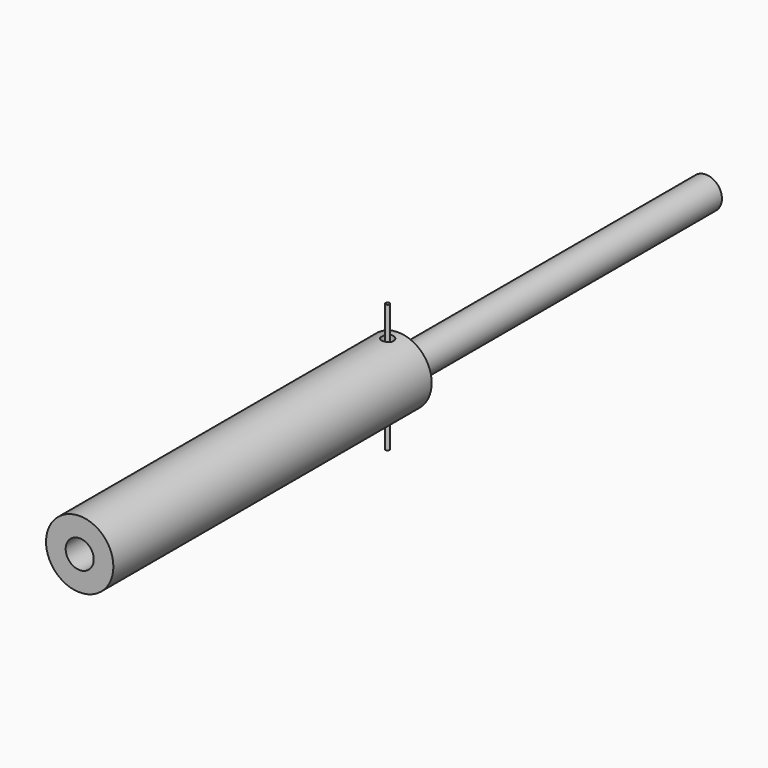
from build123d import *

# Parameters (mm, degrees)
F0_R      = 53.34
F0_R_2    = 22.225
F1_DEPTH  = 20.6375
F6_DEPTH  = 609.6
F5_R      = 9.525
F5_R_2    = 3.302
F7_DEPTH  = 19.05
F8_DEPTH  = 32.3616602869
F4_R      = 9.525
F4_R_2    = 3.302
F9_DEPTH  = 19.05
F10_DEPTH = 32.3616602869
F13_W     = 2.032
F13_H     = 3.556
F15_R     = 3.175
F16_DEPTH = 101.6
F19_R     = 25.4
F19_R_2   = 22.225
F20_DEPTH = 9.525
F21_DEPTH = 609.6


# Not quite as in the source:
# - the program builds the solid bodies; features that only make, move or delete a surface that nothing else refers to are left out


with BuildPart() as f1:
    # F0 (on Front) → F1 (new body)
    with BuildSketch(Plane.XZ):
        Circle(F0_R)
        Circle(F0_R_2, mode=Mode.SUBTRACT)
    extrude(amount=-F1_DEPTH)

    # F0 (on Front) → F6 (join)
    with BuildSketch(Plane.XZ):
        Circle(F0_R)
        Circle(F0_R_2, mode=Mode.SUBTRACT)
    extrude(amount=F6_DEPTH)

    # F5 (on offset) → F7 (cut)
    with BuildSketch(Plane.XY.offset(-53.34)):
        Circle(F5_R)
        Circle(F5_R_2, mode=Mode.SUBTRACT)
        Circle(F5_R_2)
    extrude(amount=F7_DEPTH, mode=Mode.SUBTRACT)

    # F5 (on offset) → F8 (cut, up to face)
    with BuildSketch(Plane.XY.offset(-53.34)):
        Circle(F5_R_2)
    extrude(amount=F8_DEPTH, mode=Mode.SUBTRACT)

    # F4 (on offset) → F9 (cut)
    with BuildSketch(Plane.XY.offset(53.34)):
        Circle(F4_R)
        Circle(F4_R_2, mode=Mode.SUBTRACT)
        Circle(F4_R_2)
    extrude(amount=-F9_DEPTH, mode=Mode.SUBTRACT)

    # F4 (on offset) → F10 (cut, up to face)
    with BuildSketch(Plane.XY.offset(53.34)):
        Circle(F4_R_2)
    extrude(amount=-F10_DEPTH, mode=Mode.SUBTRACT)

    # F11 (on Right) → F12 (revolve, cut)
    with BuildSketch(Plane.YZ):
        Polygon((6.35, 34.29), (3.302, 34.29), (3.302, 29.21), align=None)
        Polygon((3.302, -29.21), (3.302, -34.29), (6.35, -34.29), align=None)
    revolve(axis=Axis((0, 0, 6.9711627439), (0, 0, 1)), mode=Mode.SUBTRACT)

    # F13 (on Top) → F14 (revolve, cut)
    with BuildSketch(Plane.XY):
        Polygon((-25.4254, 11.1125), (-22.225, 11.1125), (-22.225, 20.6375), (-25.4254, 20.6375), (-25.4254, 17.653), (-25.4254, 14.097), align=None)
        with Locations((-26.4414, 15.875)):
            Rectangle(F13_W, F13_H)
    revolve(axis=Axis((0, 5.55625, 0), (0, 1, 0)), mode=Mode.SUBTRACT)


with BuildPart() as f16:
    # F15 (on Top) → F16 (new body, symmetric)
    with BuildSketch(Plane.XY):
        Circle(F15_R)
    extrude(amount=F16_DEPTH, both=True)


with BuildPart() as f20:
    # F19 (on face) → F20 (new body)
    with BuildSketch(Plane(origin=(0, 20.6375, 0), x_dir=(-1, 0, 0), z_dir=(0, 1, 0))):
        Circle(F19_R)
        Circle(F19_R_2, mode=Mode.SUBTRACT)
    extrude(amount=-F20_DEPTH)

    # F21 (add): a face of the model
    f21_faces = [f20.faces().sort_by_distance(p)[0] for p in [
        (24.6815795103, 20.6375, 0),
    ]]
    extrude(f21_faces, amount=F21_DEPTH)


solid = Compound([f1.part, f16.part, f20.part])
